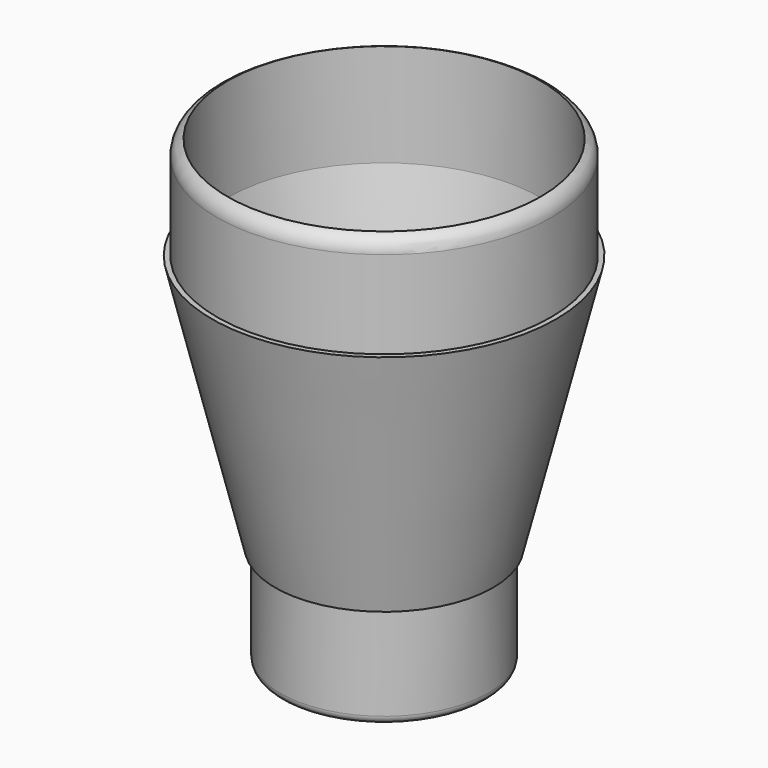
from build123d import *

# Parameters (mm, degrees)
F0_W     = 2.00000108
F0_H     = 20.0000108
F2_R     = 18.19299892
F3_DEPTH = 2.00000108
F4_R     = 1.5875


# Not quite as in the source:
# - a fillet or chamfer that OpenCascade refuses, or shapes differently, is made with other operations: its cross-section is extruded or revolved along the edge and cut away or added


with BuildPart() as f1:
    # F0 (on Front) → F1 (revolve)
    with BuildSketch(Plane.XZ):
        with Locations((19.19299946, 10.0000054)):
            Rectangle(F0_W, F0_H)
        Polygon((30.48659892, 69.9999108), (18.19299892, 20.0000108), (20.193, 20.0000108), (21.19299292, 20.0000108), (33.48659292, 69.9999108), (32.4866, 69.9999108), align=None)
        with Locations((31.48659946, 79.9999162)):
            Rectangle(F0_W, F0_H)
    revolve(axis=Axis((0, 0, 12.2811223036), (0, 0, 1)))

    # F2 (on Top) → F3 (join)
    with BuildSketch(Plane.XY):
        Circle(F2_R)
    extrude(amount=F3_DEPTH)

    # F4
    f4_edges = [f1.edges().sort_by_distance(p)[0] for p in [
        (-20.193, 0, 0),
    ]]
    fillet(f4_edges, radius=F4_R)

    # F5: fillet of radius 3.175 on 1 edges, made by hand

    # F5_s1 → F5_t2 (revolve, cut)
    with BuildSketch(Plane.XZ):
        with BuildLine():
            ThreePointArc((32.4866, 87.050344929), (31.9394552634, 88.8321983782), (30.48659892, 89.9999216))
            Line((30.48659892, 89.9999216), (32.4866, 89.9999216))
            Line((32.4866, 89.9999216), (32.4866, 87.050344929))
        make_face()
    revolve(axis=Axis((0, 0, 89.9999216), (0, 0, 1)), mode=Mode.SUBTRACT)


solid = f1.part
